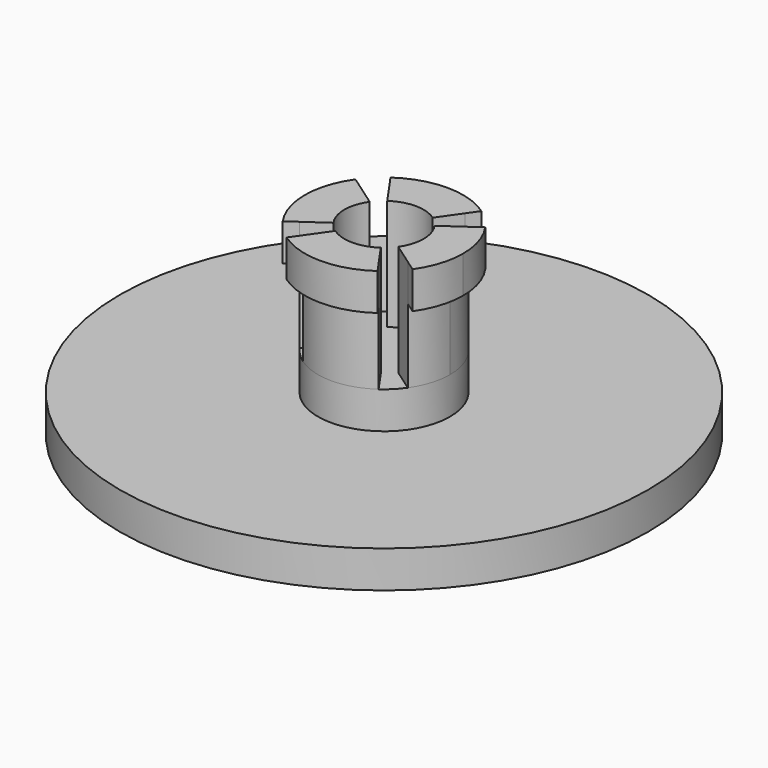
from build123d import *

# Parameters (mm, degrees)
F0_R     = 10
F1_DEPTH = 1.4
F2_R     = 2.5
F3_DEPTH = 1.4
F5_DEPTH = 2.8
F7_DEPTH = 1.4


with BuildPart() as f1:
    # F0 (on Top) → F1 (new body)
    with BuildSketch(Plane.XY):
        Circle(F0_R)
    extrude(amount=F1_DEPTH)

    # F2 (on face) → F3 (join)
    with BuildSketch(Plane.XY.offset(1.4)):
        Circle(F2_R)
    extrude(amount=F3_DEPTH)

    # F4 (on face) → F5 (join)
    with BuildSketch(Plane.XY.offset(2.8)):
        with BuildLine():
            Line((-2.0478801107, -1.4339410909), (-1.2287280664, -0.8603646545))
            ThreePointArc((-1.2287280664, -0.8603646545), (-1.5, 0), (-1.2287280664, 0.8603646545))
            Line((-1.2287280664, 0.8603646545), (-2.0478801107, 1.4339410909))
            ThreePointArc((-2.0478801107, 1.4339410909), (-2.5, 0), (-2.0478801107, -1.4339410909))
        make_face()
        with BuildLine():
            ThreePointArc((-0.8603646545, 1.2287280664), (0, 1.5), (0.8603646545, 1.2287280664))
            Line((0.8603646545, 1.2287280664), (1.4339410909, 2.0478801107))
            ThreePointArc((1.4339410909, 2.0478801107), (0, 2.5), (-1.4339410909, 2.0478801107))
            Line((-1.4339410909, 2.0478801107), (-0.8603646545, 1.2287280664))
        make_face()
        with BuildLine():
            ThreePointArc((1.2287280664, 0.8603646545), (1.4305754261, 0.4510586993), (1.5, 0))
            ThreePointArc((1.5, 0), (1.4305754261, -0.4510586993), (1.2287280664, -0.8603646545))
            Line((1.2287280664, -0.8603646545), (2.0478801107, -1.4339410909))
            ThreePointArc((2.0478801107, -1.4339410909), (2.3842923769, -0.7517644988), (2.5, 0))
            ThreePointArc((2.5, 0), (2.3842923769, 0.7517644988), (2.0478801107, 1.4339410909))
            Line((2.0478801107, 1.4339410909), (1.2287280664, 0.8603646545))
        make_face()
        with BuildLine():
            Line((1.4339410909, -2.0478801107), (0.8603646545, -1.2287280664))
            ThreePointArc((0.8603646545, -1.2287280664), (0, -1.5), (-0.8603646545, -1.2287280664))
            Line((-0.8603646545, -1.2287280664), (-1.4339410909, -2.0478801107))
            ThreePointArc((-1.4339410909, -2.0478801107), (0, -2.5), (1.4339410909, -2.0478801107))
        make_face()
    extrude(amount=F5_DEPTH)

    # F6 (on face) → F7 (join)
    with BuildSketch(Plane.XY.offset(5.6)):
        with BuildLine():
            ThreePointArc((-0.8603646545, 1.2287280664), (0, 1.5), (0.8603646545, 1.2287280664))
            Line((0.8603646545, 1.2287280664), (1.4339410909, 2.0478801107))
            ThreePointArc((1.4339410909, 2.0478801107), (0, 2.5), (-1.4339410909, 2.0478801107))
            Line((-1.4339410909, 2.0478801107), (-0.8603646545, 1.2287280664))
        make_face()
        with BuildLine():
            ThreePointArc((-1.4339410909, 2.0478801107), (0, 2.5), (1.4339410909, 2.0478801107))
            Line((1.4339410909, 2.0478801107), (1.7207293091, 2.4574561329))
            ThreePointArc((1.7207293091, 2.4574561329), (0, 3), (-1.7207293091, 2.4574561329))
            Line((-1.7207293091, 2.4574561329), (-1.4339410909, 2.0478801107))
        make_face()
        with BuildLine():
            ThreePointArc((3, 0), (2.8611508522, 0.9021173985), (2.4574561329, 1.7207293091))
            Line((2.4574561329, 1.7207293091), (2.0478801107, 1.4339410909))
            Line((2.0478801107, 1.4339410909), (1.2287280664, 0.8603646545))
            ThreePointArc((1.2287280664, 0.8603646545), (1.5, 0), (1.2287280664, -0.8603646545))
            Line((1.2287280664, -0.8603646545), (2.0478801107, -1.4339410909))
            Line((2.0478801107, -1.4339410909), (2.4574561329, -1.7207293091))
            ThreePointArc((2.4574561329, -1.7207293091), (2.8611508522, -0.9021173985), (3, 0))
        make_face()
        with BuildLine():
            Line((-2.0478801107, 1.4339410909), (-2.4574561329, 1.7207293091))
            ThreePointArc((-2.4574561329, 1.7207293091), (-3, 0), (-2.4574561329, -1.7207293091))
            Line((-2.4574561329, -1.7207293091), (-2.0478801107, -1.4339410909))
            ThreePointArc((-2.0478801107, -1.4339410909), (-2.5, 0), (-2.0478801107, 1.4339410909))
        make_face()
        with BuildLine():
            Line((-1.2287280664, 0.8603646545), (-2.0478801107, 1.4339410909))
            ThreePointArc((-2.0478801107, 1.4339410909), (-2.5, 0), (-2.0478801107, -1.4339410909))
            Line((-2.0478801107, -1.4339410909), (-1.2287280664, -0.8603646545))
            ThreePointArc((-1.2287280664, -0.8603646545), (-1.5, 0), (-1.2287280664, 0.8603646545))
        make_face()
        with BuildLine():
            Line((-1.4339410909, -2.0478801107), (-1.7207293091, -2.4574561329))
            ThreePointArc((-1.7207293091, -2.4574561329), (0, -3), (1.7207293091, -2.4574561329))
            Line((1.7207293091, -2.4574561329), (1.4339410909, -2.0478801107))
            Line((1.4339410909, -2.0478801107), (0.8603646545, -1.2287280664))
            ThreePointArc((0.8603646545, -1.2287280664), (0, -1.5), (-0.8603646545, -1.2287280664))
            Line((-0.8603646545, -1.2287280664), (-1.4339410909, -2.0478801107))
        make_face()
    extrude(amount=F7_DEPTH)


solid = f1.part
